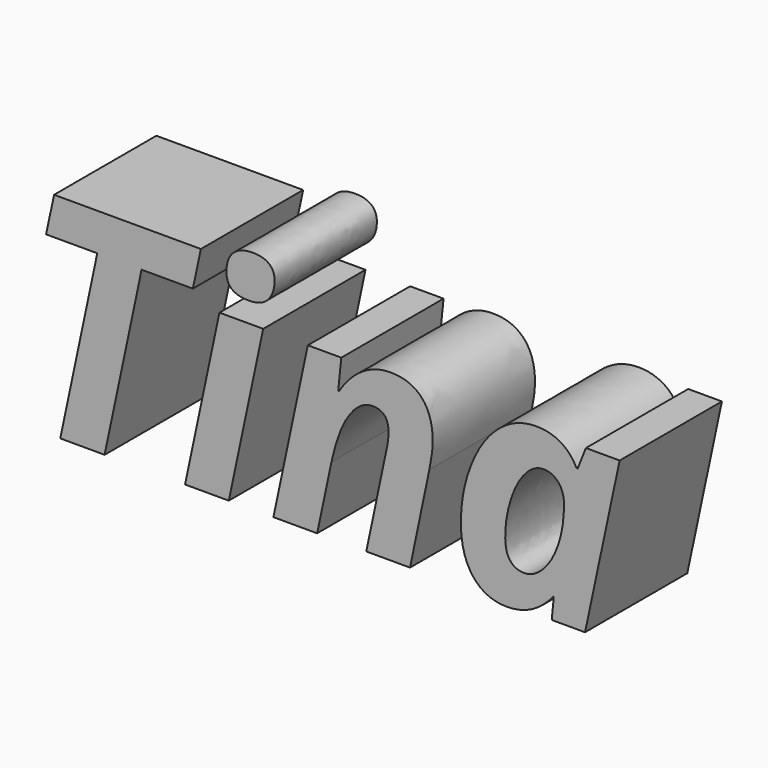
from build123d import *

# Parameters (mm, degrees)
F0_TEXT_SIZE = 59.1348572117
F1_DEPTH     = 25.4


# Not quite as in the source:
# - Text() gives the source's letters only with a copy of the font that has no kerning and outlines rounded to 1/6400 em; it was checked with that copy


with BuildPart() as f1:
    # F0 (on Front) → F1 (new body)
    with BuildSketch(Plane.XZ):
        with Locations((-65.6310096383, -27.2415950894)):
            Text('Tina', F0_TEXT_SIZE, font='Open Sans', font_style=FontStyle.BOLDITALIC, text_align=(TextAlign.LEFT, TextAlign.BOTTOM))
    extrude(amount=F1_DEPTH)


solid = f1.part
